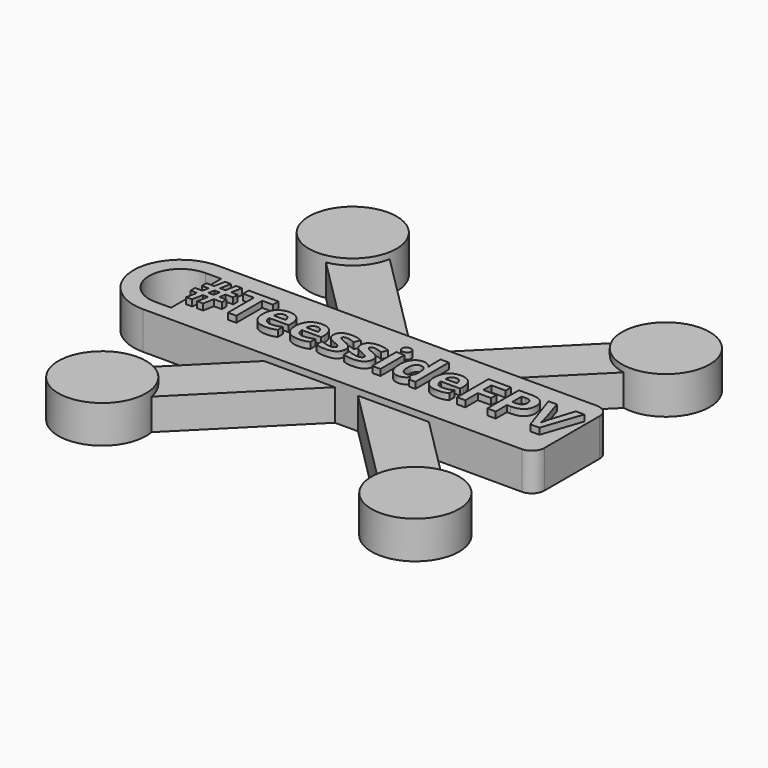
from build123d import *

# Parameters (mm, degrees)
F1_W         = 30
F1_H         = 7.5
F2_DEPTH     = 3
F1_R         = 3.5
F3_TEXT_SIZE = 4.3982223851
F4_DEPTH     = 0.5
F6_DEPTH     = 2.5
F7_DEPTH     = 5
F8_R         = 3.74999
F10_DEPTH    = 25
F11_R        = 1


# Not quite as in the source:
# - a fillet or chamfer is up to 0.001 mm smaller than in the source, because OpenCascade refuses the exact size
# - Text() gives the source's letters only with a copy of the font that has no kerning and outlines rounded to 1/6400 em; it was checked with that copy


with BuildPart() as f2:
    # F1 (on Top) → F2 (new body)
    with BuildSketch(Plane.XY):
        Rectangle(F1_W, F1_H)
    extrude(amount=F2_DEPTH)

    # F3 (on face) → F4 (join)
    with BuildSketch(Plane.XY.offset(3)):
        with Locations((-15, -1.5522687726)):
            Text('#TeessideFPV', F3_TEXT_SIZE, font='Open Sans', font_style=FontStyle.BOLD, text_align=(TextAlign.LEFT, TextAlign.BOTTOM))
    extrude(amount=F4_DEPTH)



with BuildPart() as f2b:
    # F1 (on Top) → F2, piece 2 (new body)
    with BuildSketch(Plane.XY):
        with Locations((-12.5, 12.5)):
            Circle(F1_R)
    extrude(amount=F2_DEPTH)


with BuildPart() as f2c:
    # F1 (on Top) → F2, piece 3 (new body)
    with BuildSketch(Plane.XY):
        with Locations((-12.5, -12.5)):
            Circle(F1_R)
    extrude(amount=F2_DEPTH)


with BuildPart() as f2d:
    # F1 (on Top) → F2, piece 4 (new body)
    with BuildSketch(Plane.XY):
        with Locations((12.5, -12.5)):
            Circle(F1_R)
    extrude(amount=F2_DEPTH)


with BuildPart() as f2e:
    # F1 (on Top) → F2, piece 5 (new body)
    with BuildSketch(Plane.XY):
        with Locations((12.5, 12.5)):
            Circle(F1_R)
    extrude(amount=F2_DEPTH)


with BuildPart() as f2_1:
    add(f2.part)

    add(f2b.part)  # F6 merges F2b

    add(f2c.part)  # F6 merges F2c

    add(f2d.part)  # F6 merges F2d

    add(f2e.part)  # F6 merges F2e
    # F5 (on face) → F6 (join)
    with BuildSketch(Plane(origin=(0, 0, 0), x_dir=(1, 0, 0), z_dir=(0, 0, -1))):
        Polygon((13.9142135624, 11.0857864376), (11.0857864376, 13.9142135624), (0, 2.8284271247), (2.8284271247, 0), align=None)
        Polygon((2.8284271247, 0), (0, 2.8284271247), (-2.8284271247, 0), (0, -2.8284271247), align=None)
        Polygon((-2.8284271247, 0), (0, 2.8284271247), (-11.0857864376, 13.9142135624), (-13.9142135624, 11.0857864376), align=None)
        Polygon((0, -2.8284271247), (-2.8284271247, 0), (-13.9142135624, -11.0857864376), (-11.0857864376, -13.9142135624), align=None)
        Polygon((13.9142135624, -11.0857864376), (2.8284271247, 0), (0, -2.8284271247), (11.0857864376, -13.9142135624), align=None)
    extrude(amount=-F6_DEPTH)

    # F7 (add): a face of the model
    f7_faces = [f2_1.faces().sort_by_distance(p)[0] for p in [
        (-15, 0, 1.5),
    ]]
    extrude(f7_faces, amount=F7_DEPTH)

    # F8 (radius 3.75 in the source; OpenCascade refuses exactly that, so slightly less here)
    f8_edges = [f2_1.edges().sort_by_distance(p)[0] for p in [
        (-20, 3.75, 1.5),
        (-20, -3.75, 1.5),
    ]]
    fillet(f8_edges, radius=F8_R)

    # F9 (on face) → F10 (cut)
    with BuildSketch(Plane.XY.offset(3)):
        with BuildLine():
            Line((-15, 2.5), (-16.25, 2.5))
            ThreePointArc((-16.25, 2.5), (-18.75, 0), (-16.25, -2.5))
            Line((-16.25, -2.5), (-15, -2.5))
            Line((-15, -2.5), (-15, 2.5))
        make_face()
    extrude(amount=-F10_DEPTH, mode=Mode.SUBTRACT)

    # F11
    f11_edges = [f2_1.edges().sort_by_distance(p)[0] for p in [
        (15, -3.75, 1.5),
        (15, 3.75, 1.5),
    ]]
    fillet(f11_edges, radius=F11_R)


solid = f2_1.part
